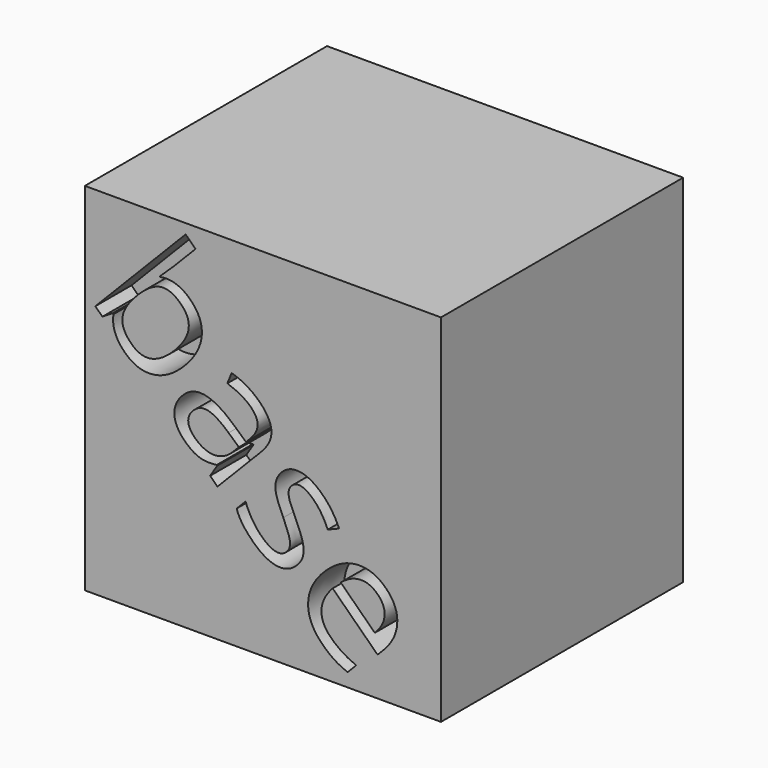
from build123d import *

# Parameters (mm, degrees)
F0_W         = 200
F0_H         = 200
F1_DEPTH     = 170
F2_TEXT_SIZE = 95.6090560654
F3_DEPTH     = 25.4


# Not quite as in the source:
# - Text() gives the source's letters only with a copy of the font that has no kerning and outlines rounded to 1/6400 em; it was checked with that copy


with BuildPart() as f1:
    # F0 (on Front) → F1 (new body)
    with BuildSketch(Plane.XZ):
        with Locations((-3932.8033575875, -2434.8270060122)):
            Rectangle(F0_W, F0_H)
    extrude(amount=F1_DEPTH)

    # F2 (on face) → F3 (cut)
    with BuildSketch(Plane.XZ.offset(170)):
        with Locations(Location((-4032.8033575875, -2386.6902525672), (0, 0, -44.2728212569))):
            Text('base', F2_TEXT_SIZE, font='Open Sans', text_align=(TextAlign.LEFT, TextAlign.BOTTOM))
    extrude(amount=-F3_DEPTH, mode=Mode.SUBTRACT)


solid = f1.part
